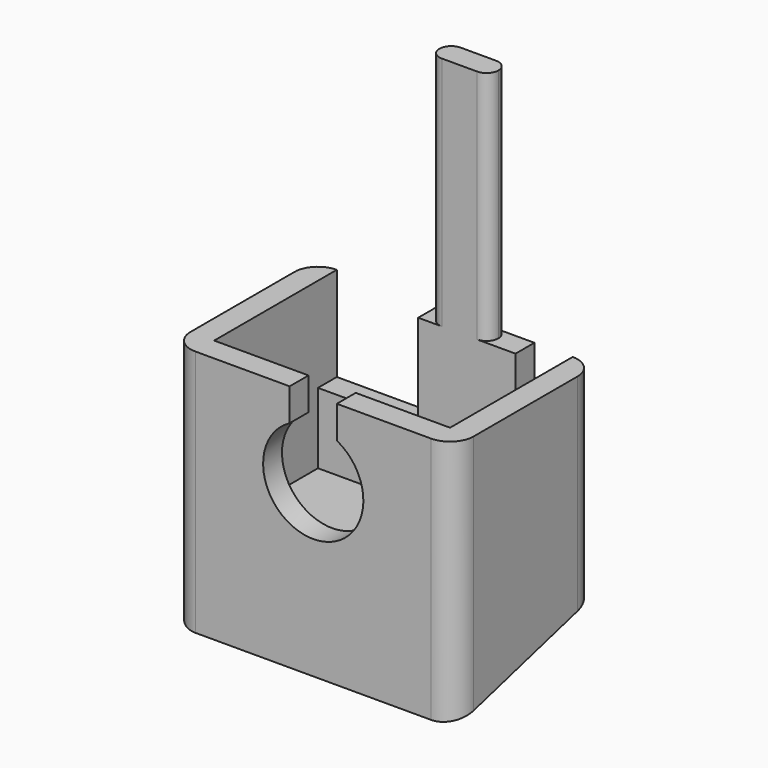
from build123d import *

# Parameters (mm, degrees)
F0_W      = 24
F0_H      = 15
F1_DEPTH  = 16
F2_T      = -2
F4_DEPTH  = 5
F5_W      = 5
F5_H      = 2
F6_DEPTH  = 20
F7_DEPTH  = 5
F9_R      = 0.99999
F10_R     = 2
F11_W     = 8.5
F11_H     = 2
F12_DEPTH = 8
F13_W     = 3.25
F13_H     = 2
F14_DEPTH = 4
F15_DEPTH = 25


# Not quite as in the source:
# - a fillet or chamfer is up to 0.001 mm smaller than in the source, because OpenCascade refuses the exact size


with BuildPart() as f1:
    # F0 (on Top) → F1 (new body)
    with BuildSketch(Plane.XY):
        Rectangle(F0_W, F0_H)
    extrude(amount=F1_DEPTH)

    # F2
    f2_openings = [f1.faces().sort_by_distance(p)[0] for p in [
        (0, 0, 16),
    ]]
    offset(amount=F2_T, openings=f2_openings)

    # F3 (on face) → F4 (cut)
    with BuildSketch(Plane.XZ.offset(7.5)):
        with BuildLine():
            Line((-2, 16), (-2, 13.25))
            ThreePointArc((-2, 13.25), (0, 5.25), (2, 13.25))
            Line((2, 13.25), (2, 16))
            Line((2, 16), (-2, 16))
        make_face()
    extrude(amount=-F4_DEPTH, mode=Mode.SUBTRACT)

    # F5 (on face) → F6 (join)
    with BuildSketch(Plane.XY.offset(16)):
        with Locations((2, 6.5)):
            Rectangle(F5_W, F5_H)
    extrude(amount=F6_DEPTH)

    # F7 (add): a face of the model
    f7_faces = [f1.faces().sort_by_distance(p)[0] for p in [
        (0, 0, 0),
    ]]
    extrude(f7_faces, amount=F7_DEPTH)

    # F9 (radius 1 in the source; OpenCascade refuses exactly that, so slightly less here)
    f9_edges = [f1.edges().sort_by_distance(p)[0] for p in [
        (4.5, 5.5, 26),
        (4.5, 7.5, 26),
        (-0.5, 5.5, 26),
        (-0.5, 7.5, 26),
    ]]
    fillet(f9_edges, radius=F9_R)

    # F10
    f10_edges = [f1.edges().sort_by_distance(p)[0] for p in [
        (12, -7.5, 5.5),
        (-12, -7.5, 5.5),
        (-12, 7.5, 5.5),
        (12, 7.5, 5.5),
    ]]
    fillet(f10_edges, radius=F10_R)

    # F11 (on face) → F12 (cut)
    with BuildSketch(Plane.XY.offset(16)):
        with Locations((-5.75, 6.5)):
            Rectangle(F11_W, F11_H)
    extrude(amount=-F12_DEPTH, mode=Mode.SUBTRACT)

    # F13 (on face) → F14 (cut)
    with BuildSketch(Plane.XY.offset(16)):
        with Locations((8.375, 6.5)):
            Rectangle(F13_W, F13_H)
    extrude(amount=-F14_DEPTH, mode=Mode.SUBTRACT)

    # F8 (on face) → F15 (cut)
    with BuildSketch(Plane.YZ.offset(12)):
        Polygon((7.5, -0.9807621135), (-7.5, -5), (7.5, -5), align=None)
    extrude(amount=-F15_DEPTH, mode=Mode.SUBTRACT)


solid = f1.part
